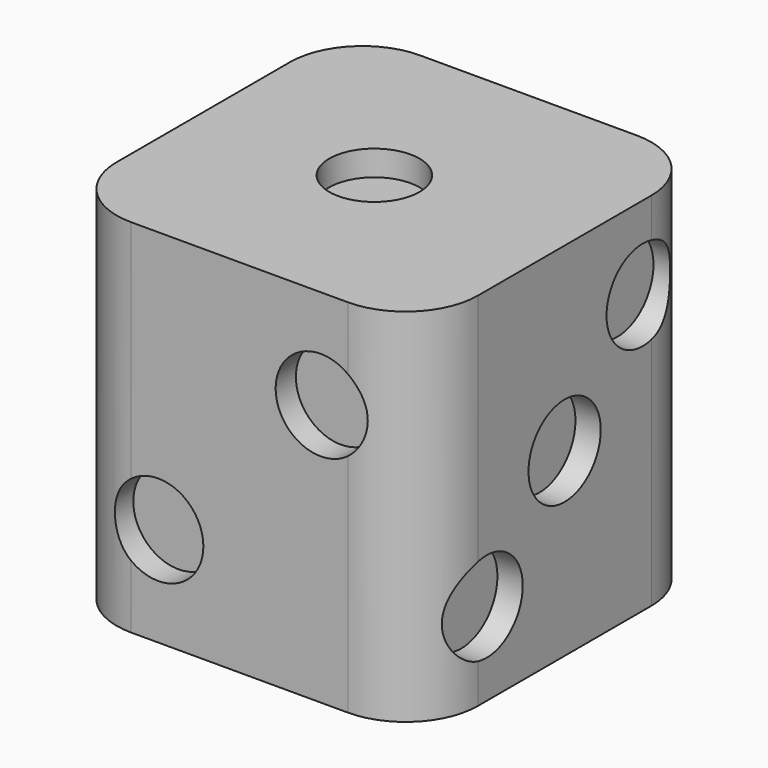
from build123d import *

# Parameters (mm, degrees)
F0_W         = 25.4
F0_H         = 25.4
F1_DEPTH     = 25.4
F2_R         = 3.175
F9_DEPTH     = 1.778
F3_R         = 3.175
F10_DEPTH    = 1.778
F4_R         = 3.175
F11_DEPTH    = 1.778
F5_R         = 3.175
F12_DEPTH    = 1.778
F6_R         = 3.175
F13_DEPTH    = 1.778
F7_R         = 3.175
F14_DEPTH    = 1.778
F8_R         = 3.175
F15_DEPTH    = 1.778
F16_T1_DEPTH = 50.8


# Not quite as in the source:
# - a fillet or chamfer that OpenCascade refuses, or shapes differently, is made with other operations: its cross-section is extruded or revolved along the edge and cut away or added


with BuildPart() as f1:
    # F0 (on Front) → F1 (new body)
    with BuildSketch(Plane.XZ):
        with Locations((-25.9571580286, 18.6469587497)):
            Rectangle(F0_W, F0_H)
    extrude(amount=F1_DEPTH)

    # F2 (on face) → F9 (cut)
    with BuildSketch(Plane.XZ.offset(25.4)):
        with Locations((-31.6721580286, 12.9319587497)):
            Circle(F2_R)
    extrude(amount=-F9_DEPTH, mode=Mode.SUBTRACT)

    # F3 (on face) → F10 (cut)
    with BuildSketch(Plane.XZ.offset(25.4)):
        with Locations((-20.2421580286, 24.3619587497)):
            Circle(F3_R)
    extrude(amount=-F10_DEPTH, mode=Mode.SUBTRACT)

    # F4 (on face) → F11 (cut)
    with BuildSketch(Plane.XY.offset(31.3469587497)):
        with Locations((-26.6341753304, -12.7)):
            Circle(F4_R)
    extrude(amount=-F11_DEPTH, mode=Mode.SUBTRACT)

    # F5 (on face) → F12 (cut)
    with BuildSketch(Plane(origin=(-38.6571580286, 0, 0), x_dir=(0, -1, 0), z_dir=(-1, 0, 0))):
        with Locations((16.7485739568, 23.0596062836)):
            Circle(F5_R)
        with Locations((16.7485739568, 14.0053418102)):
            Circle(F5_R)
        with Locations((6.985, 23.0596062836)):
            Circle(F5_R)
        with Locations((6.985, 14.0053418102)):
            Circle(F5_R)
    extrude(amount=-F12_DEPTH, mode=Mode.SUBTRACT)

    # F6 (on face) → F13 (cut)
    with BuildSketch(Plane.YZ.offset(-13.2571580286)):
        with Locations((-12.7, 18.6469587497)):
            Circle(F6_R)
        with Locations((-19.558, 11.7889587497)):
            Circle(F6_R)
        with Locations((-5.842, 25.5049587497)):
            Circle(F6_R)
    extrude(amount=-F13_DEPTH, mode=Mode.SUBTRACT)

    # F7 (on face) → F14 (cut)
    with BuildSketch(Plane(origin=(0, 0, 5.9469587497), x_dir=(1, 0, 0), z_dir=(0, 0, -1))):
        with Locations((-32.3071580286, 12.7)):
            Circle(F7_R)
        with Locations((-19.6071580286, 12.7)):
            Circle(F7_R)
        with Locations((-32.3071580286, 20.5331463367)):
            Circle(F7_R)
        with Locations((-32.3071580286, 3.81)):
            Circle(F7_R)
        with Locations((-19.6071580286, 3.81)):
            Circle(F7_R)
        with Locations((-19.6071580286, 20.8129025996)):
            Circle(F7_R)
    extrude(amount=-F14_DEPTH, mode=Mode.SUBTRACT)

    # F8 (on face) → F15 (cut)
    with BuildSketch(Plane(origin=(0, 0, 0), x_dir=(-1, 0, 0), z_dir=(0, 1, 0))):
        with Locations((25.9571580286, 19.88068223)):
            Circle(F8_R)
        with Locations((18.3371580286, 26.2669587497)):
            Circle(F8_R)
        with Locations((18.3371580286, 11.0269587497)):
            Circle(F8_R)
        with Locations((33.5771580286, 11.0269587497)):
            Circle(F8_R)
        with Locations((33.5771580286, 26.2669587497)):
            Circle(F8_R)
    extrude(amount=-F15_DEPTH, mode=Mode.SUBTRACT)

    # F16: fillet of radius 5.08 on 4 edges, made by hand

    # F16_s2 → F16_t1 (cut)
    with BuildSketch(Plane.XY.offset(-6.7530412503)):
        with BuildLine():
            ThreePointArc((-33.5771580286, -25.4), (-37.1692604771, -23.9121024484), (-38.6571580286, -20.32))
            Line((-38.6571580286, -20.32), (-38.6571580286, -25.4))
            Line((-38.6571580286, -25.4), (-33.5771580286, -25.4))
        make_face()
        with BuildLine():
            ThreePointArc((-13.2571580286, -20.32), (-14.7450555802, -23.9121024484), (-18.3371580286, -25.4))
            Line((-18.3371580286, -25.4), (-13.2571580286, -25.4))
            Line((-13.2571580286, -25.4), (-13.2571580286, -20.32))
        make_face()
        with BuildLine():
            ThreePointArc((-13.2571580286, -5.08), (-14.7450555802, -1.4878975516), (-18.3371580286, 0))
            Line((-18.3371580286, 0), (-13.2571580286, 0))
            Line((-13.2571580286, 0), (-13.2571580286, -5.08))
        make_face()
        with BuildLine():
            ThreePointArc((-33.5771580286, 0), (-37.1692604771, -1.4878975516), (-38.6571580286, -5.08))
            Line((-38.6571580286, -5.08), (-38.6571580286, 0))
            Line((-38.6571580286, 0), (-33.5771580286, 0))
        make_face()
    extrude(amount=F16_T1_DEPTH, mode=Mode.SUBTRACT)


solid = f1.part
